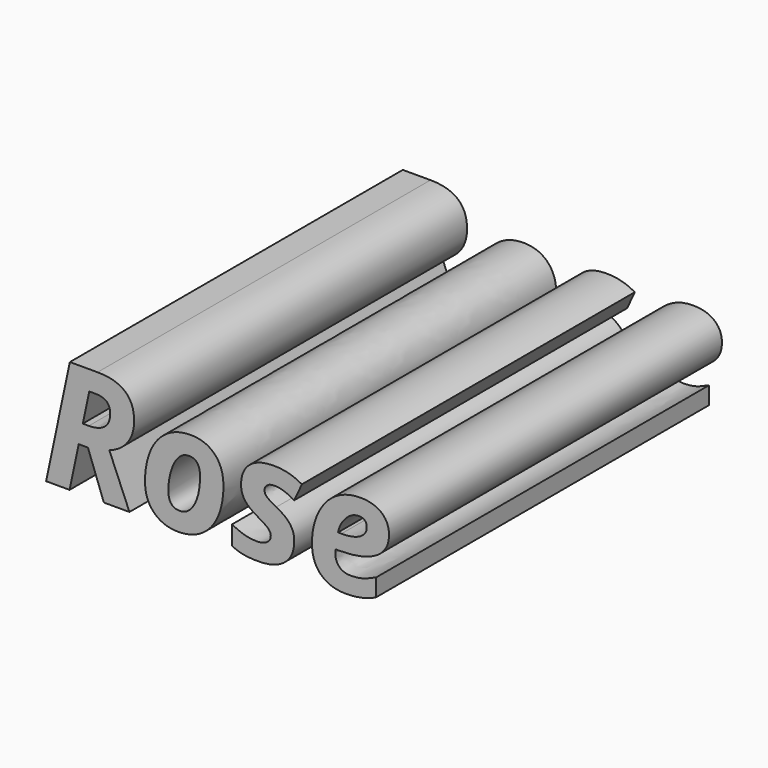
from build123d import *

# Parameters (mm, degrees)
F0_TEXT_SIZE = 9.6308335843
F1_DEPTH     = 25.4


# Not quite as in the source:
# - Text() gives the source's letters only with a copy of the font that has no kerning and outlines rounded to 1/6400 em; it was checked with that copy


with BuildPart() as f1:
    # F0 (on Front) → F1 (new body)
    with BuildSketch(Plane.XZ):
        with Locations((-14.4907003269, 2.9336998705)):
            Text('Rose', F0_TEXT_SIZE, font='Open Sans', font_style=FontStyle.BOLDITALIC, text_align=(TextAlign.LEFT, TextAlign.BOTTOM))
    extrude(amount=F1_DEPTH)


solid = f1.part
